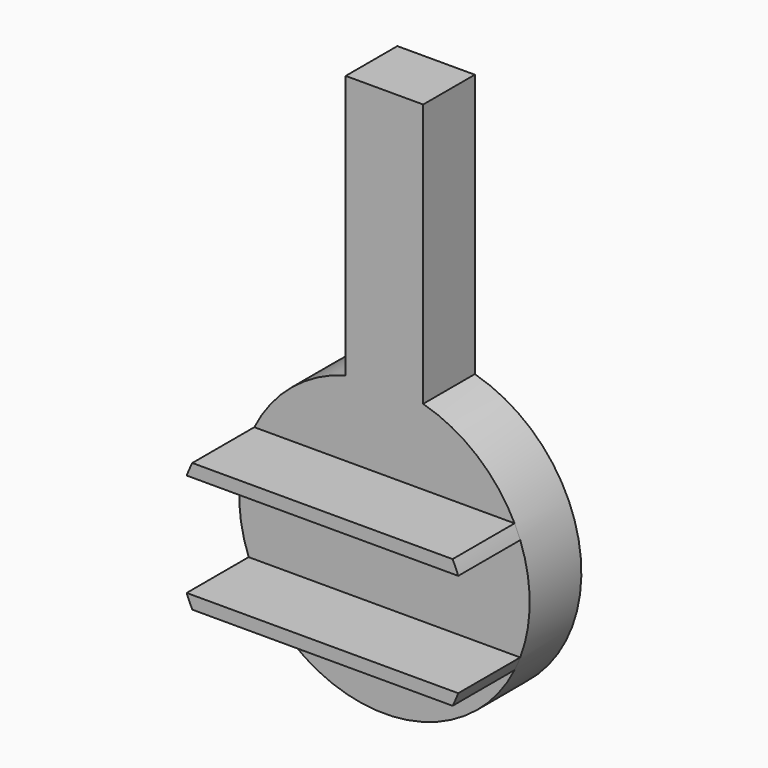
from build123d import *

# Parameters (mm, degrees)
F1_DEPTH  = 10
F2_W      = 40.3112887415
F2_H      = 2
F3_DEPTH  = 12
F6_DEPTH  = 10
F7_W      = 12
F7_H      = 10
F8_DEPTH  = 40
F9_W      = 59.6965367126
F9_H      = 7.6070292853
F10_DEPTH = 25


# Not quite as in the source:
# - a feature of the source that left no trace in its solid (it failed there, or was rolled back) is left out


with BuildPart() as f1:
    # F0 (on Front) → F1 (new body)
    with BuildSketch(Plane.XZ):
        with BuildLine():
            ThreePointArc((-6, 21.6852484422), (-13.6244265934, -17.9060045795), (22.5, 0))
            ThreePointArc((22.5, 0), (17.9060045795, 13.6244265934), (6, 21.6852484422))
            ThreePointArc((6, 21.6852484422), (3.0275328281, 22.2953816961), (0, 22.5))
            ThreePointArc((0, 22.5), (-3.0275328281, 22.2953816961), (-6, 21.6852484422))
        make_face()
    extrude(amount=F1_DEPTH)

    # F2 (on face) → F3 (join)
    with BuildSketch(Plane.XZ.offset(10)):
        with Locations((0, 9)):
            Rectangle(F2_W, F2_H)
        with Locations((0, -9)):
            Rectangle(F2_W, F2_H)
        with BuildLine():
            Line((20.1556443707, 10), (20.1556443707, 8))
            Line((20.1556443707, 8), (21.0297408448, 8))
            ThreePointArc((21.0297408448, 8), (20.6169587679, 9.0106054825), (20.1556443707, 10))
        make_face()
        with BuildLine():
            ThreePointArc((-20.1556443707, 10), (-20.6169587679, 9.0106054825), (-21.0297408448, 8))
            Line((-21.0297408448, 8), (-20.1556443707, 8))
            Line((-20.1556443707, 8), (-20.1556443707, 10))
        make_face()
        with BuildLine():
            Line((-20.1556443707, -8), (-21.0297408448, -8))
            ThreePointArc((-21.0297408448, -8), (-20.6169587679, -9.0106054825), (-20.1556443707, -10))
            Line((-20.1556443707, -10), (-20.1556443707, -8))
        make_face()
        with BuildLine():
            Line((21.0297408448, -8), (20.1556443707, -8))
            Line((20.1556443707, -8), (20.1556443707, -10))
            ThreePointArc((20.1556443707, -10), (20.6169587679, -9.0106054825), (21.0297408448, -8))
        make_face()
    extrude(amount=F3_DEPTH)

    # F0 (on Front) → F6 (join)
    with BuildSketch(Plane.XZ):
        with BuildLine():
            ThreePointArc((-6, 21.6852484422), (-13.6244265934, -17.9060045795), (22.5, 0))
            ThreePointArc((22.5, 0), (17.9060045795, 13.6244265934), (6, 21.6852484422))
            ThreePointArc((6, 21.6852484422), (3.0275328281, 22.2953816961), (0, 22.5))
            ThreePointArc((0, 22.5), (-3.0275328281, 22.2953816961), (-6, 21.6852484422))
        make_face()
        with BuildLine():
            ThreePointArc((0, 22.5), (3.0275328281, 22.2953816961), (6, 21.6852484422))
            Line((6, 21.6852484422), (6, 22.5))
            Line((6, 22.5), (0, 22.5))
        make_face()
        with BuildLine():
            Line((-6, 22.5), (-6, 21.6852484422))
            ThreePointArc((-6, 21.6852484422), (-3.0275328281, 22.2953816961), (0, 22.5))
            Line((0, 22.5), (-6, 22.5))
        make_face()
    extrude(amount=F6_DEPTH)

    # F7 (on face) → F8 (join)
    with BuildSketch(Plane.XY.offset(22.5)):
        with Locations((0, -5)):
            Rectangle(F7_W, F7_H)
    extrude(amount=F8_DEPTH)

    # F9 (on face) → F10 (cut)
    with BuildSketch(Plane.XY.offset(6)):
        with Locations((-0.8811633027, 3.8035146426)):
            Rectangle(F9_W, F9_H)
    extrude(amount=-F10_DEPTH, mode=Mode.SUBTRACT)


solid = f1.part
